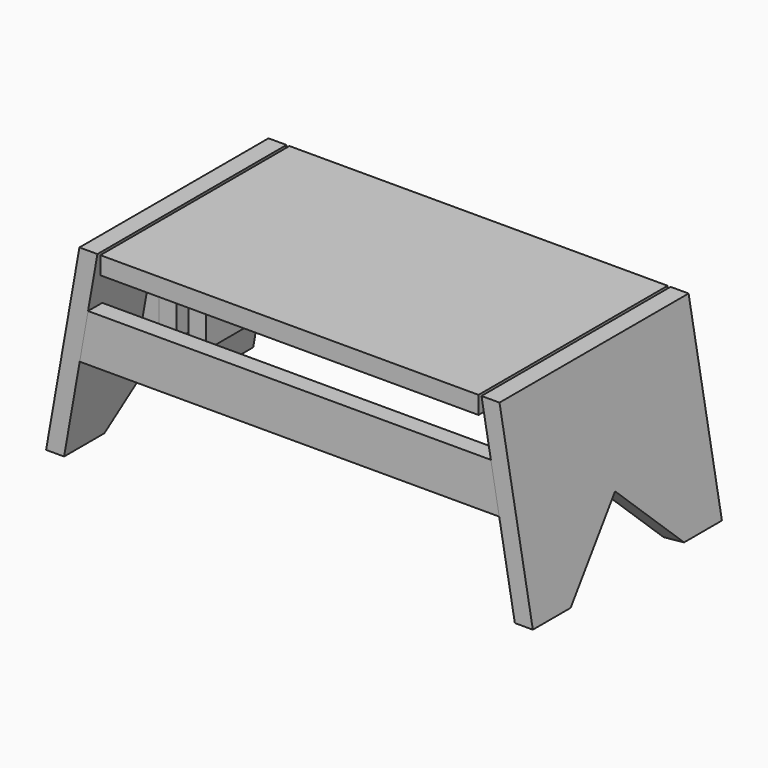
from build123d import *

# Parameters (mm, degrees)
F0_W          = 406.4
F0_H          = 254
F1_DEPTH      = 19.05
F3_DEPTH      = 127
F3_DEPTH_BACK = 127
F5_DEPTH      = 19.05
F8_DEPTH      = 19.05
F9_W          = 4.678236725
F9_H          = 12.7
F11_DEPTH     = 44.45
F10_R         = 14.2875
F10_R_2       = 12.7
F12_DEPTH     = 261.5495194364
F9_W_2        = 366.59723186
F9_W_3        = 19.05
F9_W_4        = 12.7
F9_H_2        = 36.5125
F9_H_3        = 23.8125
F9_H_4        = 1.5875
F15_DEPTH     = 44.45
F16_DEPTH     = 261.5495194364
F19_DEPTH     = 19.05
F9_H_5        = 38.1
F20_DEPTH     = 44.45
F21_DEPTH     = 261.5495194364


# Not quite as in the source:
# - a feature names something its author has since deleted; it is built from what else it names


with BuildPart() as f1:
    # F0 (on Top) → F1 (new body)
    with BuildSketch(Plane.XY):
        Rectangle(F0_W, F0_H)
    extrude(amount=F1_DEPTH)


with BuildPart() as f3:
    # F2 (on Front) → F3 (new body, two sides)
    with BuildSketch(Plane.XZ) as f3_sk:
        Polygon((261.5485194364, -184.15), (225.7188769564, 19.05), (206.375, 19.05), (242.20464248, -184.15), align=None)
    extrude(amount=F3_DEPTH)
    extrude(f3_sk.sketch, amount=-F3_DEPTH_BACK)

    # F4 (on face) → F5 (cut, through all)
    with BuildSketch(Plane(origin=(222.1703618674, 0, 39.174629111), x_dir=(0, 1, 0), z_dir=(0.984807753, 0, 0.1736481777))):
        Polygon((0, -150.5697714888), (-76.2000000001, -226.7697714888), (76.2000000001, -226.7697714888), align=None)
    extrude(amount=-F5_DEPTH, mode=Mode.SUBTRACT)


with BuildPart() as f6_1:
    # F6: instance of F3
    add(f3.part.mirror(Plane.YZ))


with BuildPart() as f8:
    # F7 (on face) → F8 (new body)
    with BuildSketch(Plane.XZ.offset(127)):
        Polygon((-216.4520869475, -38.1), (-225.4094975675, -88.9), (225.4094975675, -88.9), (216.4520869475, -38.1), align=None)
    extrude(amount=-F8_DEPTH)


with BuildPart() as f11:
    # F9 (on Front) → F11 (new body, symmetric)
    with BuildSketch(Plane.XZ):
        Polygon((-211.0377342925, -38.1), (-211.0377342925, -25.4), (-206.3594975675, -25.4), (-206.3594975675, -12.7), (-211.9733816375, -12.7), (-225.4094975675, -88.9), (-206.3594975675, -88.9), (-206.3594975675, -50.8), (-211.0377342925, -50.8), align=None)
        with Locations((-208.69861593, -31.75)):
            Rectangle(F9_W, F9_H)
        with Locations((-208.69861593, -44.45)):
            Rectangle(F9_W, F9_H)
    extrude(amount=F11_DEPTH, both=True)

    # F10 (on Right) → F12 (cut, through all)
    with BuildSketch(Plane.YZ):
        with Locations((0, -38.1)):
            Circle(F10_R)
        with Locations((0, -38.1)):
            Circle(F10_R_2, mode=Mode.SUBTRACT)
        with Locations((0, -38.1)):
            Circle(F10_R_2)
    extrude(amount=-F12_DEPTH, mode=Mode.SUBTRACT)


with BuildPart() as f13:
    # F9 (on Front) → F13 (revolve)
    with BuildSketch(Plane.XZ):
        with Locations((27.7391183625, -44.45)):
            Rectangle(F9_W_2, F9_H)
        with Locations((-208.69861593, -44.45)):
            Rectangle(F9_W, F9_H)
        with Locations((-165.0844975675, -44.45)):
            Rectangle(F9_W_3, F9_H)
        with Locations((-196.8344975675, -44.45)):
            Rectangle(F9_W_3, F9_H)
        with Locations((-180.9594975675, -44.45)):
            Rectangle(F9_W_4, F9_H)
    revolve(axis=Axis((0, 0, -38.1), (1, 0, 0)))


with BuildPart() as f14_1:
    # F14: instance of F11
    add(f11.part.mirror(Plane.YZ))


with BuildPart() as f15:
    # F9 (on Front) → F15 (new body, symmetric)
    with BuildSketch(Plane.XZ):
        with Locations((-165.0844975675, -70.64375)):
            Rectangle(F9_W_3, F9_H_2)
        with Locations((-165.0844975675, -11.90625)):
            Rectangle(F9_W_3, F9_H_3)
        with Locations((-165.0844975675, -24.60625)):
            Rectangle(F9_W_3, F9_H_4)
        with Locations((-165.0844975675, -31.75)):
            Rectangle(F9_W_3, F9_H)
        with Locations((-165.0844975675, -51.59375)):
            Rectangle(F9_W_3, F9_H_4)
        with Locations((-165.0844975675, -44.45)):
            Rectangle(F9_W_3, F9_H)
    extrude(amount=F15_DEPTH, both=True)

    # F10 (on Right) → F16 (cut, through all)
    with BuildSketch(Plane.YZ):
        with Locations((0, -38.1)):
            Circle(F10_R)
        with Locations((0, -38.1)):
            Circle(F10_R_2, mode=Mode.SUBTRACT)
        with Locations((0, -38.1)):
            Circle(F10_R_2)
    extrude(amount=-F16_DEPTH, mode=Mode.SUBTRACT)


with BuildPart() as f17_1:
    # F17: instance of F15
    add(f15.part.mirror(Plane.YZ))


with BuildPart() as f19:
    # F18 (on face) → F19 (new body)
    with BuildSketch(Plane(origin=(0, 127, 0), x_dir=(-1, 0, 0), z_dir=(0, 1, 0))):
        Polygon((209.7340289825, 0), (-209.7340289825, 0), (-218.6914396025, -50.8), (218.6914396025, -50.8), align=None)
    extrude(amount=-F19_DEPTH)


with BuildPart() as f20:
    # F9 (on Front) → F20 (new body, symmetric)
    with BuildSketch(Plane.XZ):
        with Locations((-196.8344975675, -19.05)):
            Rectangle(F9_W_3, F9_H)
        with Locations((-196.8344975675, -31.75)):
            Rectangle(F9_W_3, F9_H)
        with Locations((-196.8344975675, -44.45)):
            Rectangle(F9_W_3, F9_H)
        with Locations((-196.8344975675, -69.85)):
            Rectangle(F9_W_3, F9_H_5)
    extrude(amount=F20_DEPTH, both=True)

    # F10 (on Right) → F21 (cut, through all)
    with BuildSketch(Plane.YZ):
        with Locations((0, -38.1)):
            Circle(F10_R)
        with Locations((0, -38.1)):
            Circle(F10_R_2, mode=Mode.SUBTRACT)
        with Locations((0, -38.1)):
            Circle(F10_R_2)
    extrude(amount=-F21_DEPTH, mode=Mode.SUBTRACT)


with BuildPart() as f22_1:
    # F22: instance of F20
    add(f20.part.mirror(Plane.YZ))


solid = Compound([f1.part, f3.part, f6_1.part, f8.part, f11.part, f13.part, f14_1.part, f15.part, f17_1.part, f19.part, f20.part, f22_1.part])
